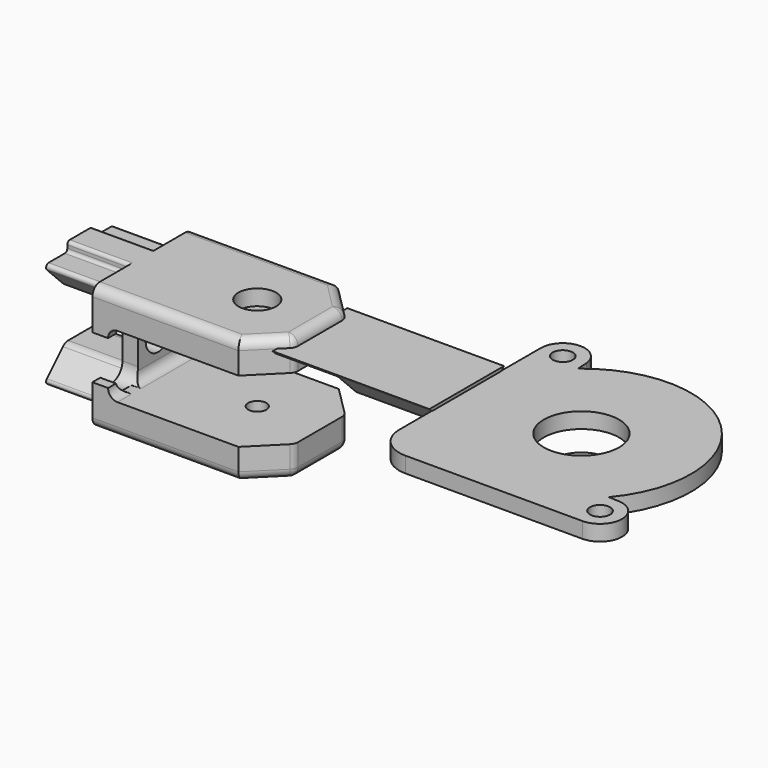
from build123d import *

# Parameters (mm, degrees)
F4_R      = 1.6
F4_R_2    = 6
F9_DEPTH  = 2.5
F5_R      = 4.5
F10_DEPTH = 6
F6_R      = 2.5
F11_DEPTH = 2.5
F12_DEPTH = 0.2
F13_DEPTH = 15
F14_DEPTH = 0.1450064733
F15_DEPTH = 25
F7_R      = 2.5
F16_DEPTH = 2.5
F17_DEPTH = 10
F8_W      = 25.8
F8_H      = 20
F8_R      = 3
F18_DEPTH = 10
F8_R_2    = 1.45
F19_DEPTH = 7.5
F20_DEPTH = 5
F21_SIZE  = 5
F22_R     = 1.49999
F22_2_R   = 1.49999
F23_F1_R  = 0.5
F23_F2_R  = 0.5
F24_R     = 5


# Not quite as in the source:
# - a fillet or chamfer is up to 0.001 mm smaller than in the source, because OpenCascade refuses the exact size


with BuildPart() as f9:
    # F4 (on Top) → F9 (new body)
    with BuildSketch(Plane.XY):
        with BuildLine():
            ThreePointArc((13.3940727278, -11.2627179563), (12.3743686708, 12.3743686708), (-11.2627179563, 13.3940727278))
            Line((-11.2627179563, 13.3940727278), (-11.3658379443, 15.2444858318))
            ThreePointArc((-11.3658379443, 15.2444858318), (-15.0443088156, 18.3495671182), (-18.3549935267, 14.8549935405))
            Line((-18.3549935267, 14.8549935405), (-18.3549935267, -18.3549935267))
            Line((-18.3549935267, -18.3549935267), (14.8549935405, -18.3549935267))
            ThreePointArc((14.8549935405, -18.3549935267), (18.3495671182, -15.0443088156), (15.2444858318, -11.3658379443))
            Line((15.2444858318, -11.3658379443), (13.3940727278, -11.2627179563))
        make_face()
        with Locations((14.8492424049, -14.8492424049)):
            Circle(F4_R, mode=Mode.SUBTRACT)
        Circle(F4_R_2, mode=Mode.SUBTRACT)
        with Locations((-14.8492424049, 14.8492424049)):
            Circle(F4_R, mode=Mode.SUBTRACT)
    extrude(amount=F9_DEPTH)

    # F6 (on offset) → F11 (join)
    with BuildSketch(Plane.YZ.offset(-18.3)):
        with BuildLine():
            Line((4, -8.4393398282), (4, -2.5606601902))
            Line((4, -2.5606601902), (6.5606601902, 0))
            Line((6.5606601902, 0), (6.9393398282, 2.5))
            Line((6.9393398282, 2.5), (2.9393398282, -1.5))
            Line((2.9393398282, -1.5), (-2.9393398282, -1.5))
            Line((-2.9393398282, -1.5), (-6.9393398282, 2.5))
            Line((-6.9393398282, 2.5), (-6.5606601902, 0))
            Line((-6.5606601902, 0), (-4, -2.5606601902))
            Line((-4, -2.5606601902), (-4, -8.4393398282))
            ThreePointArc((-4, -8.4393398282), (0, -10.4638411161), (4, -8.4393398282))
        make_face()
        with Locations((0, -5.5)):
            Circle(F6_R, mode=Mode.SUBTRACT)
        Polygon((2.9393398282, -1.5), (6.9393398282, 2.5), (-6.9393398282, 2.5), (-2.9393398282, -1.5), align=None)
    extrude(amount=F11_DEPTH)

    # F6 (on offset) → F12 (join)
    with BuildSketch(Plane.YZ.offset(-18.3)):
        with BuildLine():
            Line((4, -8.4393398282), (4, -2.5606601902))
            Line((4, -2.5606601902), (6.5606601902, 0))
            Line((6.5606601902, 0), (6.9393398282, 2.5))
            Line((6.9393398282, 2.5), (2.9393398282, -1.5))
            Line((2.9393398282, -1.5), (-2.9393398282, -1.5))
            Line((-2.9393398282, -1.5), (-6.9393398282, 2.5))
            Line((-6.9393398282, 2.5), (-6.5606601902, 0))
            Line((-6.5606601902, 0), (-4, -2.5606601902))
            Line((-4, -2.5606601902), (-4, -8.4393398282))
            ThreePointArc((-4, -8.4393398282), (0, -10.4638411161), (4, -8.4393398282))
        make_face()
        with Locations((0, -5.5)):
            Circle(F6_R, mode=Mode.SUBTRACT)
        Polygon((2.9393398282, -1.5), (6.9393398282, 2.5), (-6.9393398282, 2.5), (-2.9393398282, -1.5), align=None)
    extrude(amount=-F12_DEPTH)

    # F6 (on offset) → F13 (join)
    with BuildSketch(Plane.YZ.offset(-18.3)):
        Polygon((2.9393398282, -1.5), (6.9393398282, 2.5), (-6.9393398282, 2.5), (-2.9393398282, -1.5), align=None)
    extrude(amount=-F13_DEPTH)

    # F14 (cut, through all): a face of the model
    f14_faces = [f9.faces().sort_by_distance(p)[0] for p in [
        (-18.5, 3.8100845121, -5.5000000092),
    ]]
    extrude(f14_faces, amount=-F14_DEPTH, mode=Mode.SUBTRACT)

    # F22 (radius 1.5 in the source; OpenCascade refuses exactly that, so slightly less here)
    f22_edges = [f9.edges().sort_by_distance(p)[0] for p in [
        (-25.827497, -2.93934, -1.5),
        (-25.827497, 2.93934, -1.5),
    ]]
    fillet(f22_edges, radius=F22_R)

    # F24
    f24_edges = [f9.edges().sort_by_distance(p)[0] for p in [
        (-18.354994, -18.354994, 1.25),
    ]]
    fillet(f24_edges, radius=F24_R)


with BuildPart() as f10:
    # F5 (on offset) → F10 (new body)
    with BuildSketch(Plane.XY.offset(-2.5)):
        Circle(F5_R)
    extrude(amount=-F10_DEPTH)


with BuildPart() as f15:
    # F6 (on offset) → F15 (new body)
    with BuildSketch(Plane.YZ.offset(-18.3)):
        Polygon((-6.9393398282, 2.5), (6.9393398282, 2.5), (7.4393402533, 3.0000004619), (-7.4393402902, 3.0000004619), align=None)
    extrude(amount=-F15_DEPTH)


with BuildPart() as f16:
    # F7 (on offset) → F16 (new body)
    with BuildSketch(Plane.YZ.offset(-70)):
        with BuildLine():
            Line((-2.4999999441, -15.5), (-2.4999999441, -14.0000004619))
            Line((-2.4999999441, -14.0000004619), (-7.4393402717, -14.0000004619))
            Line((-7.4393402717, -14.0000004619), (-2.9393398098, -9.5))
            Line((-2.9393398098, -9.5), (2.9393398098, -9.5))
            Line((2.9393398098, -9.5), (7.4393402717, -14.0000004619))
            Line((7.4393402717, -14.0000004619), (2.5000000559, -14.0000004619))
            Line((2.5000000559, -14.0000004619), (2.5000000559, -15.5))
            Line((2.5000000559, -15.5), (10, -15.5))
            Line((10, -15.5), (10, -8.9999999441))
            Line((10, -8.9999999441), (8.4290278244, -8.9999999441))
            ThreePointArc((8.4290278244, -8.9999999441), (5.9674330259, -10.6715263643), (4, -8.4393398098))
            Line((4, -8.4393398282), (4, -2.5606601902))
            ThreePointArc((4, -2.5606601902), (5.9674329687, -0.328473643), (8.4290277957, -1.9999999441))
            Line((8.4290277957, -1.9999999441), (10, -1.9999999441))
            Line((10, -1.9999999441), (10, 4.5))
            Line((10, 4.5), (2.5000000559, 4.5))
            Line((2.5000000559, 4.5), (2.5000000559, 3.0000004619))
            Line((2.5000000559, 3.0000004619), (7.4393402902, 3.0000004619))
            Line((7.4393402902, 3.0000004619), (2.9393398282, -1.5))
            Line((2.9393398282, -1.5), (-2.9393398282, -1.5))
            Line((-2.9393398282, -1.5), (-7.4393402902, 3.0000004619))
            Line((-7.4393402902, 3.0000004619), (-2.4999999441, 3.0000004619))
            Line((-2.4999999441, 3.0000004619), (-2.4999999441, 4.5))
            Line((-2.4999999441, 4.5), (-10, 4.5))
            Line((-10, 4.5), (-10, -1.9999999441))
            Line((-10, -1.9999999441), (-8.4290277957, -1.9999999441))
            ThreePointArc((-8.4290277957, -1.9999999441), (-5.9674329687, -0.328473643), (-4, -2.5606601902))
            Line((-4, -2.5606601902), (-4, -8.4393398282))
            ThreePointArc((-4, -8.4393398098), (-5.9674330259, -10.6715263643), (-8.4290278244, -8.9999999441))
            Line((-8.4290278244, -8.9999999441), (-10, -8.9999999441))
            Line((-10, -8.9999999441), (-10, -15.5))
            Line((-10, -15.5), (-2.4999999441, -15.5))
        make_face()
        with Locations((0, -5.5)):
            Circle(F7_R, mode=Mode.SUBTRACT)
        Polygon((2.5000000559, 4.5), (-2.4999999441, 4.5), (-2.4999999441, 3.0000004619), (-7.4393402902, 3.0000004619), (-2.9393398282, -1.5), (2.9393398282, -1.5), (7.4393402902, 3.0000004619), (2.5000000559, 3.0000004619), align=None)
        Polygon((-7.4393402717, -14.0000004619), (-2.4999999441, -14.0000004619), (-2.4999999441, -15.5), (2.5000000559, -15.5), (2.5000000559, -14.0000004619), (7.4393402717, -14.0000004619), (2.9393398098, -9.5), (-2.9393398098, -9.5), align=None)
    extrude(amount=F16_DEPTH)

    # F7 (on offset) → F17 (join)
    with BuildSketch(Plane.YZ.offset(-70)):
        Polygon((2.5000000559, 4.5), (-2.4999999441, 4.5), (-2.4999999441, 3.0000004619), (-7.4393402902, 3.0000004619), (-2.9393398282, -1.5), (2.9393398282, -1.5), (7.4393402902, 3.0000004619), (2.5000000559, 3.0000004619), align=None)
        Polygon((-7.4393402717, -14.0000004619), (-2.4999999441, -14.0000004619), (-2.4999999441, -15.5), (2.5000000559, -15.5), (2.5000000559, -14.0000004619), (7.4393402717, -14.0000004619), (2.9393398098, -9.5), (-2.9393398098, -9.5), align=None)
    extrude(amount=-F17_DEPTH)

    # F8 (on offset) → F18 (join, symmetric)
    with BuildSketch(Plane.XY.offset(-5.5)):
        with Locations((-54.6, 0)):
            Rectangle(F8_W, F8_H)
        with Locations((-51.7, 0)):
            Circle(F8_R, mode=Mode.SUBTRACT)
    extrude(amount=F18_DEPTH, both=True)

    # F8 (on offset) → F19 (join, symmetric)
    with BuildSketch(Plane.XY.offset(-5.5)):
        with Locations((-51.7, 0)):
            Circle(F8_R)
        with Locations((-51.7, 0)):
            Circle(F8_R_2, mode=Mode.SUBTRACT)
    extrude(amount=F19_DEPTH, both=True)

    # F8 (on offset) → F20 (cut, symmetric)
    with BuildSketch(Plane.XY.offset(-5.5)):
        with Locations((-54.6, 0)):
            Rectangle(F8_W, F8_H)
        with Locations((-51.7, 0)):
            Circle(F8_R, mode=Mode.SUBTRACT)
        with Locations((-51.7, 0)):
            Circle(F8_R)
        with Locations((-51.7, 0)):
            Circle(F8_R_2, mode=Mode.SUBTRACT)
    extrude(amount=F20_DEPTH, both=True, mode=Mode.SUBTRACT)

    # F21
    f21_edges = [f16.edges().sort_by_distance(p)[0] for p in [
        (-41.7, -10, -13),
        (-41.7, 10, -13),
        (-41.7, -10, 2),
        (-41.7, 10, 2),
    ]]
    chamfer(f21_edges, length=F21_SIZE)

    # F22#2 (radius 1.5 in the source; OpenCascade refuses exactly that, so slightly less here)
    f22_2_edges = [f16.edges().sort_by_distance(p)[0] for p in [
        (-75, 2.93934, -1.5),
        (-75, -2.93934, -1.5),
        (-75, 2.93934, -9.5),
        (-75, -2.93934, -9.5),
        (-58.35, 10, 4.5),
        (-58.35, 10, -15.5),
        (-58.35, -10, -15.5),
        (-58.35, -10, 4.5),
        (-41.7, -5, -13),
        (-41.7, 5, -13),
        (-41.7, -5, 2),
        (-41.7, 5, 2),
        (-67.5, 0, -0.5),
        (-67.5, 0, -10.5),
        (-67.5, -8.576714, -10.5),
        (-67.5, -8.576714, -0.5),
        (-67.5, 8.576714, -0.5),
        (-67.5, 8.576714, -10.5),
        (-44.2, 7.5, -15.5),
        (-41.7, 0, -15.5),
        (-44.2, -7.5, -15.5),
        (-44.2, 7.5, 4.5),
        (-41.7, 0, 4.5),
        (-44.2, -7.5, 4.5),
    ]]
    fillet(f22_2_edges, radius=F22_2_R)

    # F23: fillet of radius 0.5 on 22 edges, made by hand

    # F23_f1
    f23_f1_edges = [f16.edges().sort_by_distance(p)[0] for p in [
        (-75, 7.4393402717, -14.0000004619),
        (-75, -7.4393402717, -14.0000004619),
        (-75, -2.4999999441, -15.5),
        (-75, 2.5000000559, -15.5),
        (-75, -7.4393402902, 3.0000004619),
        (-75, 7.4393402902, 3.0000004619),
        (-75, 2.5000000559, 4.5),
        (-75, -2.4999999441, 4.5),
    ]]
    fillet(f23_f1_edges, radius=F23_F1_R)

    # F23_f2
    f23_f2_edges = [f16.edges().sort_by_distance(p)[0] for p in [
        (-75, 2.5000000559, 3.0000004619),
        (-75, -2.4999999441, 3.0000004619),
        (-75, -2.4999999441, -14.0000004619),
        (-75, 2.5000000559, -14.0000004619),
        (-70, 0, -9.5),
        (-70, 0, -1.5),
        (-70, -4.9822318135, 0.5428919853),
        (-70, -2.8920449485, -1.38582006),
        (-70, 2.8920449485, -1.38582006),
        (-70, 4.9822318135, 0.5428919853),
        (-70, -4.9822317951, -11.5428919853),
        (-70, -2.8920449301, -9.61417994),
        (-70, 2.8920449301, -9.61417994),
        (-70, 4.9822317951, -11.5428919853),
        (-70, 6.6941732568, -13.6913421781),
        (-70, -6.6941732568, -13.6913421781),
        (-70, 6.6941732752, 2.6913421781),
        (-70, -6.6941732752, 2.6913421781),
    ]]
    fillet(f23_f2_edges, radius=F23_F2_R)


solid = Compound([f9.part, f10.part, f15.part, f16.part])
